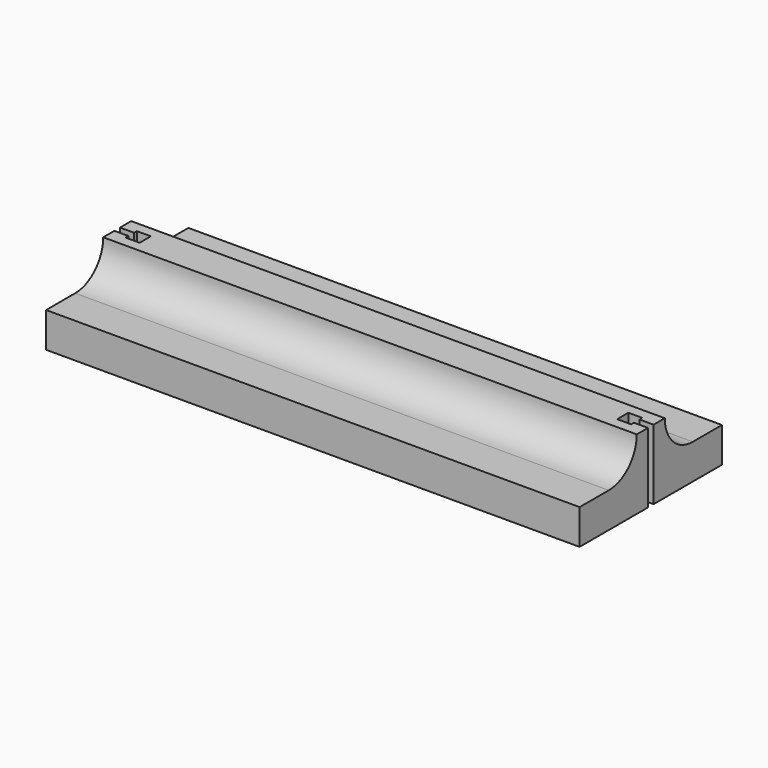
from build123d import *

# Parameters (mm, degrees)
F0_W     = 76.2
F0_H     = 25.4
F1_DEPTH = 5
F2_W     = 76.2
F2_H     = 5
F3_DEPTH = 5
F4_R     = 4.99999
F5_W     = 2
F5_H     = 2
F7_DEPTH = 2
F6_W     = 3
F6_H     = 1
F8_DEPTH = 10.001


# Not quite as in the source:
# - a fillet or chamfer is up to 0.001 mm smaller than in the source, because OpenCascade refuses the exact size


with BuildPart() as f1:
    # F0 (on Top) → F1 (new body)
    with BuildSketch(Plane.XY):
        Rectangle(F0_W, F0_H)
    extrude(amount=F1_DEPTH)

    # F2 (on face) → F3 (join)
    with BuildSketch(Plane.XY.offset(5)):
        Rectangle(F2_W, F2_H)
    extrude(amount=F3_DEPTH)

    # F4 (radius 5 in the source; OpenCascade refuses exactly that, so slightly less here)
    f4_edges = [f1.edges().sort_by_distance(p)[0] for p in [
        (0, -2.5, 5),
        (0, 2.5, 5),
    ]]
    fillet(f4_edges, radius=F4_R)

    # F5 (on face) → F7 (cut)
    with BuildSketch(Plane.XY.offset(10)):
        with Locations((35.1, 0)):
            Rectangle(F5_W, F5_H)
        with Locations((-35.1, 0)):
            Rectangle(F5_W, F5_H)
    extrude(amount=-F7_DEPTH, mode=Mode.SUBTRACT)

    # F6 (on face) → F8 (cut, through all)
    with BuildSketch(Plane.XY.offset(10)):
        with Locations((36.6, 0)):
            Rectangle(F6_W, F6_H)
        with Locations((-36.6, 0)):
            Rectangle(F6_W, F6_H)
    extrude(amount=-F8_DEPTH, mode=Mode.SUBTRACT)


solid = f1.part
